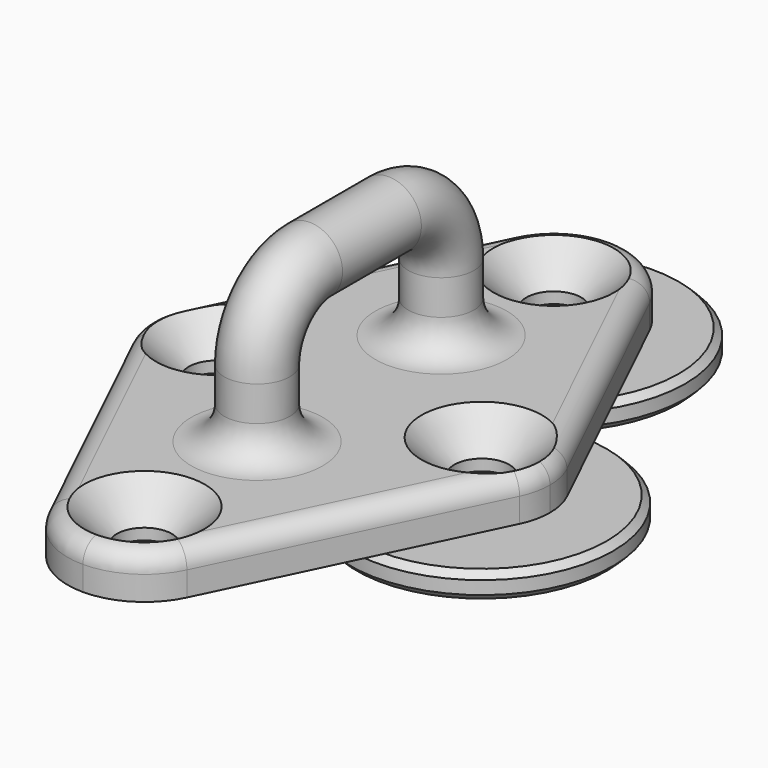
from build123d import *

# Parameters (mm, degrees)
F0_R       = 4.175
F1_DEPTH   = 6.7
F2_R       = 3
F5_R       = 5
F7_R       = 5
F9_START   = 1
F8_R       = 20
F8_R_2     = 4.175
F9_DEPTH   = 4
F10_SIZE   = 1
F10_2_SIZE = 1


# Not quite as in the source:
# - a fillet or chamfer that OpenCascade refuses, or shapes differently, is made with other operations: its cross-section is extruded or revolved along the edge and cut away or added


with BuildPart() as f1:
    # F0 (on Top) → F1 (new body)
    with BuildSketch(Plane.XY):
        with BuildLine():
            ThreePointArc((-10.5191429835, -43.989904332), (-6.2117979251, -48.810301793), (0, -50.6))
            ThreePointArc((0, -50.6), (6.2117979251, -48.810301793), (10.5191429835, -43.989904332))
            Line((10.5191429835, -43.989904332), (29.5328465485, -4.5009321151))
            ThreePointArc((29.5328465485, -4.5009321151), (30.2999526183, -2.3083237489), (30.56, 0))
            ThreePointArc((30.56, 0), (30.2999526183, 2.3083237489), (29.5328465485, 4.5009321151))
            Line((29.5328465485, 4.5009321151), (10.5191429835, 43.989904332))
            ThreePointArc((10.5191429835, 43.989904332), (6.2117979251, 48.810301793), (0, 50.6))
            ThreePointArc((0, 50.6), (-6.2117979251, 48.810301793), (-10.5191429835, 43.989904332))
            Line((-10.5191429835, 43.989904332), (-29.5328465485, 4.5009321151))
            ThreePointArc((-29.5328465485, 4.5009321151), (-30.2999526183, 2.3083237489), (-30.56, 0))
            ThreePointArc((-30.56, 0), (-30.2999526183, -2.3083237489), (-29.5328465485, -4.5009321151))
            Line((-29.5328465485, -4.5009321151), (-10.5191429835, -43.989904332))
        make_face()
        with Locations((0, -38.925)):
            Circle(F0_R, mode=Mode.SUBTRACT)
        with Locations((-20.185, 0)):
            Circle(F0_R, mode=Mode.SUBTRACT)
        with Locations((20.185, 0)):
            Circle(F0_R, mode=Mode.SUBTRACT)
        with Locations((0, 38.925)):
            Circle(F0_R, mode=Mode.SUBTRACT)
    extrude(amount=F1_DEPTH)

    # F2
    f2_edges = [f1.edges().sort_by_distance(p)[0] for p in [
        (-20.025995, -24.245418, 6.7),
        (0, -50.6, 6.7),
        (20.025995, -24.245418, 6.7),
        (20.025995, 24.245418, 6.7),
        (0, 50.6, 6.7),
        (-20.025995, 24.245418, 6.7),
    ]]
    fillet(f2_edges, radius=F2_R)

    # F3: chamfer of 5 on 4 edges, made by hand

    # F3_s1 → F3_t2 (revolve, cut)
    with BuildSketch(Plane.XZ.offset(38.925)):
        Polygon((9.175, 6.7), (4.175, 1.7), (4.175, 6.7), align=None)
    revolve(axis=Axis((0, -38.925, 6.7), (0, 0, 1)), mode=Mode.SUBTRACT)

    # F3_s3 → F3_t4 (revolve, cut)
    with BuildSketch(Plane.XZ):
        Polygon((-11.01, 6.7), (-16.01, 1.7), (-16.01, 6.7), align=None)
    revolve(axis=Axis((-20.185, 0, 6.7), (0, 0, 1)), mode=Mode.SUBTRACT)

    # F3_s5 → F3_t6 (revolve, cut)
    with BuildSketch(Plane.XZ.offset(-38.925)):
        Polygon((9.175, 6.7), (4.175, 1.7), (4.175, 6.7), align=None)
    revolve(axis=Axis((0, 38.925, 6.7), (0, 0, 1)), mode=Mode.SUBTRACT)

    # F3_s7 → F3_t8 (revolve, cut)
    with BuildSketch(Plane.XZ):
        Polygon((29.36, 6.7), (24.36, 1.7), (24.36, 6.7), align=None)
    revolve(axis=Axis((20.185, 0, 6.7), (0, 0, 1)), mode=Mode.SUBTRACT)

    # F6: sweep along a path in F4
    with BuildLine(Plane.YZ) as f6_path:
        Line((-17.5, 0), (-17.5, 17))
        ThreePointArc((-17.5, 17), (-14.5710678119, 24.0710678119), (-7.5, 27))
        Line((-7.5, 27), (0, 27))
        Line((0, 27), (7.5, 27))
        ThreePointArc((7.5, 27), (14.5710678119, 24.0710678119), (17.5, 17))
        Line((17.5, 17), (17.5, 0))
    # F5 (on Top) → F6 (sweep)
    with BuildSketch(Plane.XY):
        with Locations((0, -17.5)):
            Circle(F5_R)
    sweep(path=f6_path.line)

    # F7
    f7_edges = [f1.edges().sort_by_distance(p)[0] for p in [
        (-5, -17.5, 6.7),
        (-5, 17.5, 6.7),
    ]]
    fillet(f7_edges, radius=F7_R)


with BuildPart() as f9:
    # F8 (on face) → F9 (new body)
    with BuildSketch(Plane(origin=(0, 0, 0), x_dir=(1, 0, 0), z_dir=(0, 0, -1)).offset(F9_START)):
        with Locations((0, -38.925)):
            Circle(F8_R)
        with Locations((0, -38.925)):
            Circle(F8_R_2, mode=Mode.SUBTRACT)
    extrude(amount=F9_DEPTH)

    # F10
    f10_edges = [f9.edges().sort_by_distance(p)[0] for p in [
        (-20, 38.925, -5),
        (-4.175, 38.925, -5),
        (-20, 38.925, -1),
    ]]
    chamfer(f10_edges, length=F10_SIZE)


with BuildPart() as f9b:
    # F8 (on face) → F9, piece 2 (new body)
    with BuildSketch(Plane(origin=(0, 0, 0), x_dir=(1, 0, 0), z_dir=(0, 0, -1)).offset(F9_START)):
        with Locations((20.185, 0)):
            Circle(F8_R)
        with Locations((20.185, 0)):
            Circle(F8_R_2, mode=Mode.SUBTRACT)
    extrude(amount=F9_DEPTH)

    # F10#2
    f10_2_edges = [f9b.edges().sort_by_distance(p)[0] for p in [
        (0.185, 0, -5),
        (0.185, 0, -1),
    ]]
    chamfer(f10_2_edges, length=F10_2_SIZE)


solid = Compound([f1.part, f9.part, f9b.part])
